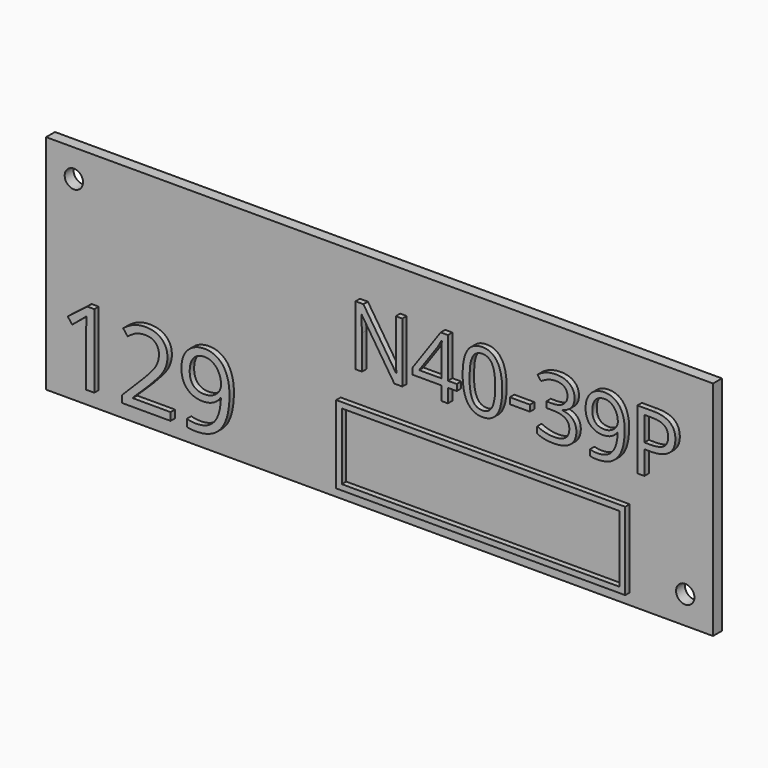
from build123d import *

# Parameters (mm, degrees)
F0_W         = 120
F0_H         = 40
F1_DEPTH     = 2
F3_D         = 3.3
F4_TEXT_SIZE = 15.0824823252
F5_DEPTH     = 1
F6_TEXT_SIZE = 18.5356140827
F7_DEPTH     = 1
F8_W         = 52
F8_H         = 14
F8_W_2       = 49.99999962
F8_H_2       = 11.99999962
F9_DEPTH     = 1


# Not quite as in the source:
# - Text() gives the source's letters only with a copy of the font that has no kerning and outlines rounded to 1/6400 em; it was checked with that copy


with BuildPart() as f1:
    # F0 (on Front) → F1 (new body)
    with BuildSketch(Plane.XZ):
        Rectangle(F0_W, F0_H)
    extrude(amount=F1_DEPTH)

    # F3 (through all)
    with Locations(Plane.XZ.offset(2)):
        with Locations((-55, 15), (55, -15)):
            Hole(F3_D / 2)

    # F4 (on face) → F5 (join)
    with BuildSketch(Plane.XZ.offset(2)):
        with Locations((-5, 2)):
            Text('N40-39P', F4_TEXT_SIZE, font='Open Sans', text_align=(TextAlign.LEFT, TextAlign.BOTTOM))
    extrude(amount=F5_DEPTH)

    # F6 (on face) → F7 (join)
    with BuildSketch(Plane.XZ.offset(2)):
        with Locations((-57, -17)):
            Text('129', F6_TEXT_SIZE, font='Open Sans', text_align=(TextAlign.LEFT, TextAlign.BOTTOM))
    extrude(amount=F7_DEPTH)

    # F8 (on face) → F9 (join)
    with BuildSketch(Plane.XZ.offset(2)):
        with Locations((19, -11)):
            Rectangle(F8_W, F8_H)
        with Locations((19, -11)):
            Rectangle(F8_W_2, F8_H_2, mode=Mode.SUBTRACT)
    extrude(amount=F9_DEPTH)


solid = f1.part
